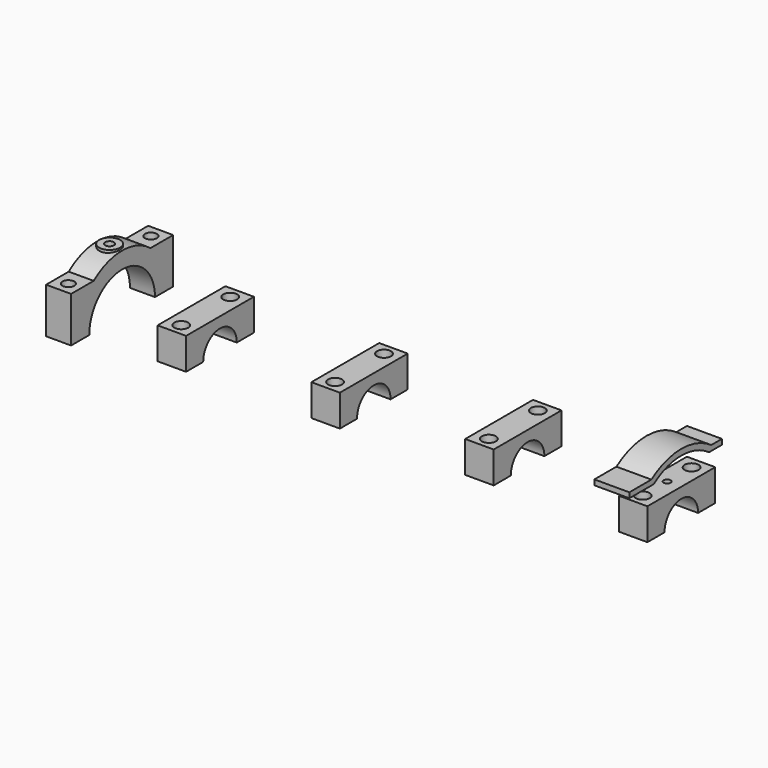
from build123d import *

# Parameters (mm, degrees)
F2_DEPTH       = 39.1
F0_R           = 4
F0_R_2         = 3.4
F3_DEPTH       = 11
F4_R           = 12
F5_DEPTH       = 334.25
F6_R           = 23.5
F7_DEPTH       = 14.3
F8_W           = 39.7
F8_H           = 15.3
F8_W_2         = 71.7
F8_W_3         = 71.75
F9_DEPTH       = 53.75
F22_DEPTH      = 514
F16_R          = 24.75
F23_DEPTH      = 39.7
F17_R          = 25
F24_DEPTH      = 71.7
F18_R          = 25
F25_DEPTH      = 71.7
F19_R          = 25
F26_DEPTH      = 71.75
F28_DEPTH      = 18
F30_R          = 50
F30_R_2        = 30.8
F31_DEPTH      = 319.95
F32_END_RADIUS = 30.8
F15_R          = 6.5
F15_R_2        = 6
F32_REACH      = 57.4857763109
F0_R_3         = 2.5
F0_R_4         = 3
F0_R_5         = 2
F33_DEPTH      = 39.1010001
F35_DEPTH      = 20
F36_W          = 116.0697114092
F36_H          = 45.8095933202
F37_DEPTH      = 319.95
F38_W          = 39.7
F38_H          = 22.9808008298
F38_W_2        = 71.7
F38_H_2        = 22.1049790271
F38_H_3        = 21.3201404549
F38_W_3        = 71.75
F38_H_4        = 20.5597863533
F39_DEPTH      = 7.001
F39_DEPTH_BACK = 66.6798368476
F40_R          = 4
F41_DEPTH      = 10.1
F42_R          = 10
F43_DEPTH      = 5


# Not quite as in the source:
# - an extrude ends at something that could not be found from the text; its depth is read off the source's solid


with BuildPart() as f2:
    # F1 (on Top) → F2 (new body)
    with BuildSketch(Plane.XY):
        Polygon((7.15, 7), (-7.15, 7), (-7.15, -66), (7.15, -66), (7.15, -53.75), (327.1, -53.75), (327.1, -5.25), (7.15, -5.25), align=None)
    extrude(amount=F2_DEPTH)

    # F0 (on Top) → F3 (cut)
    with BuildSketch(Plane.XY):
        with Locations((55, -12)):
            Circle(F0_R)
        with Locations((55, -12)):
            Circle(F0_R_2, mode=Mode.SUBTRACT)
        with Locations((231, -12)):
            Circle(F0_R)
        with Locations((231, -12)):
            Circle(F0_R_2, mode=Mode.SUBTRACT)
    extrude(amount=F3_DEPTH, mode=Mode.SUBTRACT)

    # F4 (on face) → F5 (cut, through all)
    with BuildSketch(Plane.YZ.offset(327.1)):
        with Locations((-29.5, 0)):
            Circle(F4_R)
    extrude(amount=-F5_DEPTH, mode=Mode.SUBTRACT)

    # F6 (on face) → F7 (cut)
    with BuildSketch(Plane(origin=(-7.15, 0, 0), x_dir=(0, -1, 0), z_dir=(-1, 0, 0))):
        with Locations((29.5, 0)):
            Circle(F6_R)
    extrude(amount=-F7_DEPTH, mode=Mode.SUBTRACT)

    # F8 (on Front) → F9 (cut, through all)
    with BuildSketch(Plane.XZ):
        with Locations((27, 7.65)):
            Rectangle(F8_W, F8_H)
        with Locations((99, 7.65)):
            Rectangle(F8_W_2, F8_H)
        with Locations((187, 7.65)):
            Rectangle(F8_W_2, F8_H)
        with Locations((275.025, 7.65)):
            Rectangle(F8_W_3, F8_H)
    extrude(amount=F9_DEPTH, mode=Mode.SUBTRACT)

    # F21 (on offset) → F22 (cut, through all)
    with BuildSketch(Plane(origin=(-7.15, 0, 0), x_dir=(0, -1, 0), z_dir=(-1, 0, 0))):
        with BuildLine():
            ThreePointArc((9.1775985671, 26), (29.5, 33), (49.8224014329, 26))
            Line((49.8224014329, 26), (66, 26))
            Line((66, 26), (66, 39.1))
            Line((66, 39.1), (-7, 39.1))
            Line((-7, 39.1), (-7, 26))
            Line((-7, 26), (9.1775985671, 26))
        make_face()
    extrude(amount=-F22_DEPTH, mode=Mode.SUBTRACT)

    # F16 (on offset) → F23 (cut, through all)
    with BuildSketch(Plane.YZ.offset(7.15)):
        with Locations((-29.5, 0)):
            Circle(F16_R)
    extrude(amount=F23_DEPTH, mode=Mode.SUBTRACT)

    # F17 (on offset) → F24 (cut, through all)
    with BuildSketch(Plane.YZ.offset(63.15)):
        with Locations((-29.5, 0)):
            Circle(F17_R)
    extrude(amount=F24_DEPTH, mode=Mode.SUBTRACT)

    # F18 (on offset) → F25 (cut, through all)
    with BuildSketch(Plane.YZ.offset(151.15)):
        with Locations((-29.5, 0)):
            Circle(F18_R)
    extrude(amount=F25_DEPTH, mode=Mode.SUBTRACT)

    # F19 (on offset) → F26 (cut, through all)
    with BuildSketch(Plane.YZ.offset(239.15)):
        with Locations((-29.5, 0)):
            Circle(F19_R)
    extrude(amount=F26_DEPTH, mode=Mode.SUBTRACT)

    # F27 (on face) → F28 (cut)
    with BuildSketch(Plane.XY.offset(39.1)):
        with BuildLine():
            Line((63.1, -59), (63.1, -47))
            ThreePointArc((63.1, -47), (55, -38.9), (46.9, -47))
            Line((46.9, -47), (46.9, -59))
            Line((46.9, -59), (63.1, -59))
        make_face()
        with BuildLine():
            Line((63.1, -12), (63.1, 0))
            Line((63.1, 0), (46.9, 0))
            Line((46.9, 0), (46.9, -12))
            ThreePointArc((46.9, -12), (55, -20.1), (63.1, -12))
        make_face()
        with BuildLine():
            Line((151.1, -12), (151.1, 0))
            Line((151.1, 0), (134.9, 0))
            Line((134.9, 0), (134.9, -12))
            ThreePointArc((134.9, -12), (143, -20.1), (151.1, -12))
        make_face()
        with BuildLine():
            Line((151.1, -59), (151.1, -47))
            ThreePointArc((151.1, -47), (143, -38.9), (134.9, -47))
            Line((134.9, -47), (134.9, -59))
            Line((134.9, -59), (151.1, -59))
        make_face()
        with BuildLine():
            Line((239.1, -12), (239.1, 0))
            Line((239.1, 0), (222.9, 0))
            Line((222.9, 0), (222.9, -12))
            ThreePointArc((222.9, -12), (231, -20.1), (239.1, -12))
        make_face()
        with BuildLine():
            Line((239.1, -59), (239.1, -47))
            ThreePointArc((239.1, -47), (231, -38.9), (222.9, -47))
            Line((222.9, -47), (222.9, -59))
            Line((222.9, -59), (239.1, -59))
        make_face()
        with BuildLine():
            ThreePointArc((310.9, -12), (319, -20.1), (327.1, -12))
            Line((327.1, -12), (327.1, 0))
            Line((327.1, 0), (310.9, 0))
            Line((310.9, 0), (310.9, -12))
        make_face()
        with BuildLine():
            Line((327.1, -59), (327.1, -47))
            ThreePointArc((327.1, -47), (319, -38.9), (310.9, -47))
            Line((310.9, -47), (310.9, -59))
            Line((310.9, -59), (327.1, -59))
        make_face()
    extrude(amount=-F28_DEPTH, mode=Mode.SUBTRACT)

    # F30 (on offset) → F31 (cut, through all)
    with BuildSketch(Plane.YZ.offset(327.1)):
        with Locations((-29.5, 0)):
            Circle(F30_R)
        with Locations((-29.5, 0)):
            Circle(F30_R_2, mode=Mode.SUBTRACT)
    extrude(amount=-F31_DEPTH, mode=Mode.SUBTRACT)

    f32_end = (Plane(origin=(167.125, -29.5, 0), x_dir=(0, 0, 1), z_dir=(1, 0, 0)) * Cylinder(F32_END_RADIUS, 802.4046404691, mode=Mode.PRIVATE)).faces().sort_by_distance((167.125, -29.5, 30.8))[0]
    # F15 (on offset) → F32 (join, up to the whole of a round face its end follows)
    with BuildSketch(Plane.XY.offset(39.1)):
        with Locations((27.5, -22)):
            Circle(F15_R)
        with Locations((162.5, -22)):
            Circle(F15_R)
        with Locations((298.5, -22)):
            Circle(F15_R)
        with Locations((0, -29.5)):
            Circle(F15_R_2)
    f32_long = extrude(amount=-F32_REACH, mode=Mode.PRIVATE)
    add(split(f32_long, bisect_by=f32_end, keep=Keep.TOP, mode=Mode.PRIVATE))

    # F0 (on Top) → F33 (cut, through all)
    with BuildSketch(Plane.XY):
        Circle(F0_R_2)
        with Locations((143, -12)):
            Circle(F0_R_2)
        with Locations((319, -12)):
            Circle(F0_R_2)
        with Locations((231, -47)):
            Circle(F0_R_2)
        with Locations((319, -47)):
            Circle(F0_R_2)
        with Locations((143, -47)):
            Circle(F0_R_2)
        with Locations((55, -47)):
            Circle(F0_R_2)
        with Locations((0, -59)):
            Circle(F0_R_2)
        with Locations((0, -29.5)):
            Circle(F0_R_3)
        with Locations((27.5, -22)):
            Circle(F0_R_4)
        with Locations((162.5, -22)):
            Circle(F0_R_4)
        with Locations((298.5, -22)):
            Circle(F0_R_4)
        with Locations((55, -12)):
            Circle(F0_R_2)
        with Locations((231, -12)):
            Circle(F0_R_2)
        with Locations((319, -29.5)):
            Circle(F0_R_5)
    extrude(amount=F33_DEPTH, mode=Mode.SUBTRACT)

    # F36 (on offset) → F37 (cut, through all)
    with BuildSketch(Plane.YZ.offset(327.1)):
        with Locations((-27.0535778254, 41.0047966601)):
            Rectangle(F36_W, F36_H)
    extrude(amount=-F37_DEPTH, mode=Mode.SUBTRACT)

    # F38 (on Front) → F39 (cut, two sides)
    with BuildSketch(Plane.XZ) as f39_sk:
        with Locations((27, 11.4904004149)):
            Rectangle(F38_W, F38_H)
        with Locations((99, 11.0524895135)):
            Rectangle(F38_W_2, F38_H_2)
        with Locations((187, 10.6600702275)):
            Rectangle(F38_W_2, F38_H_3)
        with Locations((275.025, 10.2798931766)):
            Rectangle(F38_W_3, F38_H_4)
    extrude(amount=-F39_DEPTH, mode=Mode.SUBTRACT)
    extrude(f39_sk.sketch, amount=F39_DEPTH_BACK, mode=Mode.SUBTRACT)

    # F40 (on face) → F41 (cut)
    with BuildSketch(Plane.XY.offset(18.1)):
        with Locations((55, -12)):
            Circle(F40_R)
        with Locations((143, -12)):
            Circle(F40_R)
        with Locations((231, -12)):
            Circle(F40_R)
        with Locations((319, -12)):
            Circle(F40_R)
        with Locations((319, -47)):
            Circle(F40_R)
        with Locations((231, -47)):
            Circle(F40_R)
        with Locations((143, -47)):
            Circle(F40_R)
        with Locations((55, -47)):
            Circle(F40_R)
    extrude(amount=-F41_DEPTH, mode=Mode.SUBTRACT)

    # F42 (on offset) → F43 (cut)
    with BuildSketch(Plane.XY.offset(39.1)):
        with Locations((0, -29.5)):
            Circle(F42_R)
    extrude(amount=-F43_DEPTH, mode=Mode.SUBTRACT)


with BuildPart() as f35:
    # F34 (on offset) → F35 (new body)
    with BuildSketch(Plane.YZ.offset(327.1)):
        with BuildLine():
            ThreePointArc((-49.290907003, 27.4), (-29.5, 33.8), (-9.709092997, 27.4))
            Line((-9.709092997, 27.4), (-0.4580076056, 27.4))
            Line((-0.4580076056, 27.4), (-0.4580076056, 30.4))
            Line((-0.4580076056, 30.4), (-8.0965911747, 30.4))
            ThreePointArc((-8.0965911747, 30.4), (-29.5, 37.1788368476), (-50.9034088253, 30.4))
            Line((-50.9034088253, 30.4), (-66.6788368476, 30.4))
            Line((-66.6788368476, 30.4), (-66.6788368476, 27.4))
            Line((-66.6788368476, 27.4), (-49.290907003, 27.4))
        make_face()
    extrude(amount=-F35_DEPTH)


solid = Compound([f2.part, f35.part])
